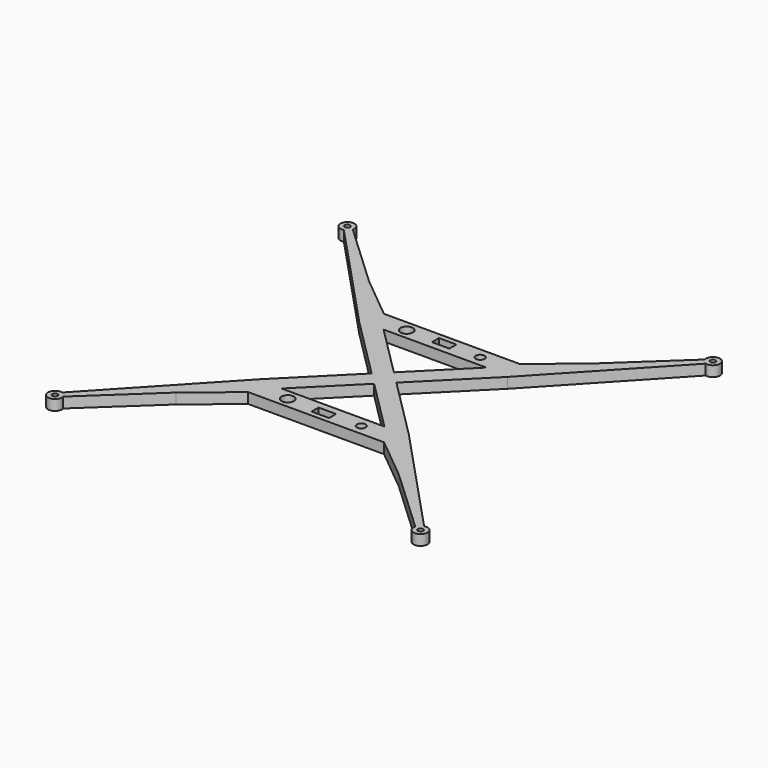
from build123d import *

# Parameters (mm, degrees)
F0_R         = 4
F1_DEPTH     = 6
F3_DEPTH     = 6
F4_R         = 1.5
F5_DEPTH     = 6.001
F6_COUNT     = 4
F8_W         = 85
F8_H         = 12
F9_DEPTH     = 6
F10_R        = 3.55
F10_R_2      = 2.5
F10_W        = 10
F10_H        = 5
F11_DEPTH    = 6.001
F12_C1_SIZE2 = 3
F12_C1_SIZE  = 30
F12_C2_SIZE2 = 30
F12_C2_SIZE  = 3
F12_C3_SIZE2 = 3
F12_C3_SIZE  = 30
F12_C4_SIZE2 = 30
F12_C4_SIZE  = 3


# Not quite as in the source:
# - a pattern or mirror of a feature is missing from the dataset's text; its kind, count and spacing are read off the source's solid


with BuildPart() as f1:
    # F0 (on Top) → F1 (new body)
    with BuildSketch(Plane.XY):
        with Locations((-104.5, 104.5)):
            Circle(F0_R)
    extrude(amount=F1_DEPTH)

    # F2 (on Top) → F3 (join, through all)
    with BuildSketch(Plane.XY):
        Polygon((-7.0710678119, 0), (0, 0), (0, 7.0710678119), (-35.3553390593, 42.4264068712), (-100.6362966948, 103.4647238196), (-103.4647238196, 100.6362966948), (-42.4264068712, 35.3553390593), align=None)
    extrude(amount=F3_DEPTH)

    # F4 (on face) → F5 (cut, through all)
    with BuildSketch(Plane.XY.offset(6)):
        with Locations((-104.5, 104.5)):
            Circle(F4_R)
    extrude(amount=-F5_DEPTH, mode=Mode.SUBTRACT)


with BuildPart() as f6_1:
    # F6: instance of F1
    add(f1.part.rotate(Axis((0, 0, 3), (0, 0, -1)), 1 * 360 / F6_COUNT))


with BuildPart() as f6_2:
    # F6: instance of F1
    add(f1.part.rotate(Axis((0, 0, 3), (0, 0, -1)), 2 * 360 / F6_COUNT))


with BuildPart() as f6_3:
    # F6: instance of F1
    add(f1.part.rotate(Axis((0, 0, 3), (0, 0, -1)), 3 * 360 / F6_COUNT))


with BuildPart() as f1_1:
    add(f1.part)

    # F7: union F6_1, F6_2, F6_3
    add(f6_1.part)
    add(f6_2.part)
    add(f6_3.part)

    # F8 (on Top) → F9 (join, through all)
    with BuildSketch(Plane.XY):
        with Locations((0, 42.5)):
            Rectangle(F8_W, F8_H)
    f9 = extrude(amount=F9_DEPTH)

    # F9_copies: F9 across plane
    add(f9.mirror(Plane(origin=(0, 0, 0), x_dir=(0, 0, -1), z_dir=(0, -1, 0))))

    # F10 (on face) → F11 (cut, through all)
    with BuildSketch(Plane.XY.offset(6)):
        with Locations((-21, 42.5)):
            Circle(F10_R)
        with Locations((21, 42.5)):
            Circle(F10_R_2)
        with Locations((0, 43)):
            Rectangle(F10_W, F10_H)
    f11 = extrude(amount=-F11_DEPTH, mode=Mode.SUBTRACT)

    # F11_copies: F11 across plane
    add(f11.mirror(Plane(origin=(0, 0, 0), x_dir=(0, 0, -1), z_dir=(0, -1, 0))), mode=Mode.SUBTRACT)

    # F12: chamfer of 3 x 30 on 4 edges, made by hand

    # F12_c1
    f12_c1_edges = [f1_1.edges().sort_by_distance(p)[0] for p in [
        (-41.8510944399, 48.5, 3),
    ]]
    f12_c1_side = f1_1.faces().sort_by_distance((-41.8949210948, 48.5409783396, 3))[0]
    chamfer(f12_c1_edges, length=F12_C1_SIZE, length2=F12_C1_SIZE2, reference=f12_c1_side)

    # F12_c2
    f12_c2_edges = [f1_1.edges().sort_by_distance(p)[0] for p in [
        (41.8510944399, 48.5, 3),
    ]]
    f12_c2_side = f1_1.faces().sort_by_distance((41.7910944399, 48.5, 3))[0]
    chamfer(f12_c2_edges, length=F12_C2_SIZE, length2=F12_C2_SIZE2, reference=f12_c2_side)

    # F12_c3
    f12_c3_edges = [f1_1.edges().sort_by_distance(p)[0] for p in [
        (41.8510944399, -48.5, 3),
    ]]
    f12_c3_side = f1_1.faces().sort_by_distance((41.8949210948, -48.5409783396, 3))[0]
    chamfer(f12_c3_edges, length=F12_C3_SIZE, length2=F12_C3_SIZE2, reference=f12_c3_side)

    # F12_c4
    f12_c4_edges = [f1_1.edges().sort_by_distance(p)[0] for p in [
        (-41.8510944399, -48.5, 3),
    ]]
    f12_c4_side = f1_1.faces().sort_by_distance((-41.7910944399, -48.5, 3))[0]
    chamfer(f12_c4_edges, length=F12_C4_SIZE, length2=F12_C4_SIZE2, reference=f12_c4_side)


solid = f1_1.part
